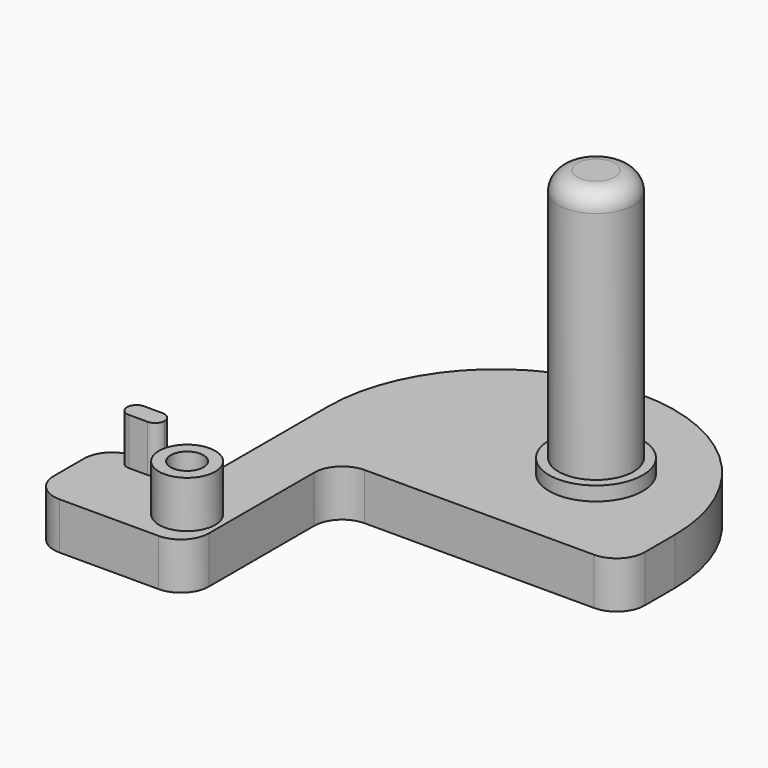
from build123d import *

# Parameters (mm, degrees)
F0_R      = 5
F0_R_2    = 1.75
F0_W      = 10
F0_H      = 10
F0_R_3    = 4
F1_DEPTH  = 5
F2_DEPTH  = 1.5
F3_R      = 4
F4_DEPTH  = 27
F5_R      = 2
F6_R      = 18
F7_R      = 3
F7_R_2    = 1.75
F8_DEPTH  = 5
F9_R      = 3
F10_W     = 4
F10_H     = 2
F11_DEPTH = 5
F12_R     = 0.99999


# Not quite as in the source:
# - a fillet or chamfer is up to 0.001 mm smaller than in the source, because OpenCascade refuses the exact size


with BuildPart() as f1:
    # F0 (on Top) → F1 (new body)
    with BuildSketch(Plane.XY):
        Polygon((-25, 15.5), (-18.459414942, 15.5), (12, 15.5), (12, 40.5), (-25, 40.5), align=None)
        with Locations((0, 27)):
            Circle(F0_R, mode=Mode.SUBTRACT)
        Polygon((-25, 5.5), (-25, -4.5), (-18.459414942, -4.5), (-18.459414942, 15.5), (-25, 15.5), align=None)
        with Locations((-22, 0)):
            Circle(F0_R_2, mode=Mode.SUBTRACT)
        with Locations((-30, 0.5)):
            Rectangle(F0_W, F0_H)
        with Locations((0, 27)):
            Circle(F0_R)
        with Locations((0, 27)):
            Circle(F0_R_3, mode=Mode.SUBTRACT)
        with Locations((0, 27)):
            Circle(F0_R_3)
    extrude(amount=-F1_DEPTH)

    # F0 (on Top) → F2 (join)
    with BuildSketch(Plane.XY):
        with Locations((0, 27)):
            Circle(F0_R)
        with Locations((0, 27)):
            Circle(F0_R_3, mode=Mode.SUBTRACT)
        with Locations((0, 27)):
            Circle(F0_R_3)
    extrude(amount=F2_DEPTH)

    # F3 (on face) → F4 (join)
    with BuildSketch(Plane.XY.offset(1.5)):
        with Locations((0, 27)):
            Circle(F3_R)
    extrude(amount=F4_DEPTH)

    # F5
    f5_edges = [f1.edges().sort_by_distance(p)[0] for p in [
        (-4, 27, 28.5),
    ]]
    fillet(f5_edges, radius=F5_R)

    # F6
    f6_edges = [f1.edges().sort_by_distance(p)[0] for p in [
        (-25, 40.5, -2.5),
        (12, 40.5, -2.5),
    ]]
    fillet(f6_edges, radius=F6_R)

    # F7 (on face) → F8 (join)
    with BuildSketch(Plane.XY):
        with Locations((-22, 0)):
            Circle(F7_R)
        with Locations((-22, 0)):
            Circle(F7_R_2, mode=Mode.SUBTRACT)
    extrude(amount=F8_DEPTH)

    # F9
    f9_edges = [f1.edges().sort_by_distance(p)[0] for p in [
        (-25, 5.5, -2.5),
        (-35, 5.5, -2.5),
        (-35, -4.5, -2.5),
        (-18.459415, -4.5, -2.5),
        (-18.459415, 15.5, -2.5),
        (12, 15.5, -2.5),
    ]]
    fillet(f9_edges, radius=F9_R)

    # F10 (on face) → F11 (join)
    with BuildSketch(Plane.XY):
        with Locations((-30, 4.5)):
            Rectangle(F10_W, F10_H)
    extrude(amount=F11_DEPTH)

    # F12 (radius 1 in the source; OpenCascade refuses exactly that, so slightly less here)
    f12_edges = [f1.edges().sort_by_distance(p)[0] for p in [
        (-32, 5.5, 2.5),
        (-32, 3.5, 2.5),
        (-28, 3.5, 2.5),
        (-28, 5.5, 2.5),
    ]]
    fillet(f12_edges, radius=F12_R)


solid = f1.part
